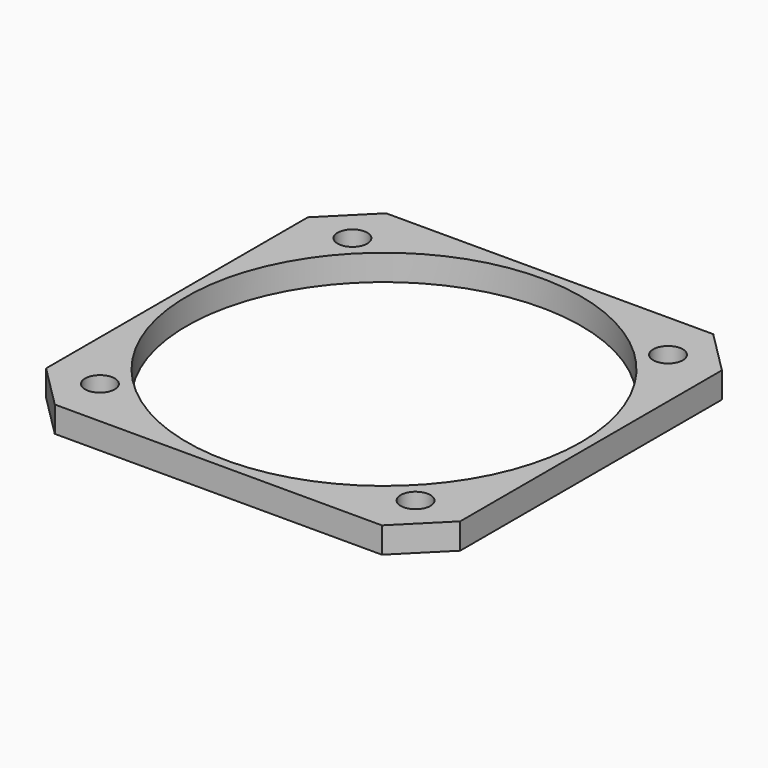
from build123d import *

# Parameters (mm, degrees)
F0_R     = 1.5
F0_R_2   = 19.9517
F1_DEPTH = 2.6162


with BuildPart() as f1:
    # F0 (on Top) → F1 (new body)
    with BuildSketch(Plane.XY):
        Polygon((-16.5498495616, -20.9517), (16.5498495616, -20.9517), (20.9517, -16.5498495616), (20.9517, 16.5498495616), (16.5498495616, 20.9517), (-16.5498495616, 20.9517), (-20.9517, 16.5498495616), (-20.9517, -16.5498495616), align=None)
        with Locations((-15.9668953833, -15.9668953833)):
            Circle(F0_R, mode=Mode.SUBTRACT)
        with Locations((15.9668953833, -15.9668953833)):
            Circle(F0_R, mode=Mode.SUBTRACT)
        with Locations((-15.9668953833, 15.9668953833)):
            Circle(F0_R, mode=Mode.SUBTRACT)
        Circle(F0_R_2, mode=Mode.SUBTRACT)
        with Locations((15.9668953833, 15.9668953833)):
            Circle(F0_R, mode=Mode.SUBTRACT)
    extrude(amount=F1_DEPTH)


solid = f1.part
